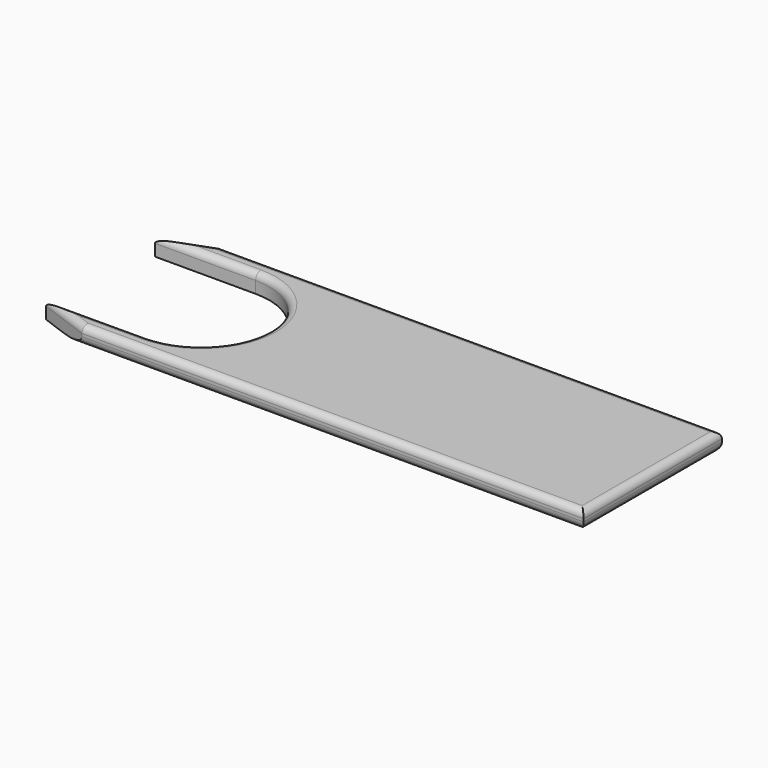
from build123d import *

# Parameters (mm, degrees)
F0_W         = 60
F0_H         = 18.8
F2_DEPTH     = 2
F3_DEPTH     = 3
F5_T1_DEPTH  = 30.5361420581
F6_SIZE2     = 5.494945
F6_SIZE      = 1.99999
F7_T1_DEPTH  = 59.3887824638
F7_T3_DEPTH  = 59.3938374638
F7_T5_DEPTH  = 22.4213203436
F7_T7_DEPTH  = 10.7363912706
F7_T9_DEPTH  = 3.6213303413
F7_T11_DEPTH = 12.745712209
F7_T13_DEPTH = 10.7363785984
F7_T15_DEPTH = 12.740667054
F7_T18_ANGLE = 180
F8_R         = 0.9656854249


# Not quite as in the source:
# - a fillet or chamfer that OpenCascade refuses, or shapes differently, is made with other operations: its cross-section is extruded or revolved along the edge and cut away or added
# - a fillet or chamfer is up to 0.001 mm smaller than in the source, because OpenCascade refuses the exact size


with BuildPart() as f2:
    # F0 (on Top) → F2 (new body)
    with BuildSketch(Plane.XY):
        Rectangle(F0_W, F0_H)
    extrude(amount=F2_DEPTH)


with BuildPart() as f3:
    # F1 (on Top) → F3 (new body)
    with BuildSketch(Plane.XY):
        with BuildLine():
            ThreePointArc((-19.0649479628, -7.3999999978), (-13.832357782, -5.2325901785), (-11.6649479628, 2.2e-09))
            ThreePointArc((-11.6649479628, 2.2e-09), (-13.832357782, 5.232590183), (-19.0649479628, 7.4000000022))
            Line((-19.0649479628, 7.4000000022), (-19.0649479628, -7.3999999978))
        make_face()
        with BuildLine():
            Line((-19.0649479628, -7.3999999978), (-19.0649479628, 7.4000000022))
            ThreePointArc((-19.0649479628, 7.4000000022), (-26.4649479628, 2.2e-09), (-19.0649479628, -7.3999999978))
        make_face()
        with BuildLine():
            ThreePointArc((-19.0649479628, -7.3999999978), (-26.4649479628, 2.2e-09), (-19.0649479628, 7.4000000022))
            Line((-19.0649479628, 7.4000000022), (-58.9926913381, 7.4000000022))
            Line((-58.9926913381, 7.4000000022), (-58.9926913381, -7.3999999978))
            Line((-58.9926913381, -7.3999999978), (-19.0649479628, -7.3999999978))
        make_face()
    extrude(amount=F3_DEPTH)


with BuildPart() as f2_1:
    add(f2.part)

    # F4: cut F3
    add(f3.part, mode=Mode.SUBTRACT)

    # F5: chamfer of 5.5 x 2.0018362885 on 1 edges, made by hand

    # F5_s2 → F5_t1 (cut)
    with BuildSketch(Plane.XY.offset(-14.268071029)):
        Polygon((-24.5, -9.4), (-30, -7.3981637115), (-30, -9.4), align=None)
    extrude(amount=F5_T1_DEPTH, mode=Mode.SUBTRACT)

    # F6 (size 2 and 5.4949548389 in the source; OpenCascade refuses exactly that, so slightly less here)
    f6_edges = [f2_1.edges().sort_by_distance(p)[0] for p in [
        (-30, 9.4, 1),
    ]]
    f6_side = f2_1.faces().sort_by_distance((-30, 8.4, 1))[0]
    chamfer(f6_edges, length=F6_SIZE, length2=F6_SIZE2, reference=f6_side)

    # F7: fillet of radius 0.7242640687 on 9 edges, made by hand

    # F7_s2 → F7_t1 (cut)
    with BuildSketch(Plane.YZ.offset(-27.578122292)):
        with BuildLine():
            ThreePointArc((-8.6757359313, 2), (-9.1878679656, 1.7878679656), (-9.4, 1.2757359313))
            Line((-9.4, 1.2757359313), (-9.4, 2))
            Line((-9.4, 2), (-8.6757359313, 2))
        make_face()
    extrude(amount=F7_T1_DEPTH, mode=Mode.SUBTRACT)

    # F7_s4 → F7_t3 (cut)
    with BuildSketch(Plane.YZ.offset(-27.583177292)):
        with BuildLine():
            ThreePointArc((9.4, 1.2757359313), (9.1878679656, 1.7878679656), (8.6757359313, 2))
            Line((8.6757359313, 2), (9.4, 2))
            Line((9.4, 2), (9.4, 1.2757359313))
        make_face()
    extrude(amount=F7_T3_DEPTH, mode=Mode.SUBTRACT)

    # F7_s6 → F7_t5 (cut)
    with BuildSketch(Plane.XZ.offset(-11.2106601718)):
        with BuildLine():
            ThreePointArc((30, 1.2757359313), (29.7878679656, 1.7878679656), (29.2757359313, 2))
            Line((29.2757359313, 2), (30, 2))
            Line((30, 2), (30, 1.2757359313))
        make_face()
    extrude(amount=F7_T5_DEPTH, mode=Mode.SUBTRACT)

    # F7_s8 → F7_t7 (cut)
    with BuildSketch(Plane(origin=(-25.8093615097, 9.3938393551, 0), x_dir=(0, 0, 1), z_dir=(0.9396926208, -0.3420201433, 0))):
        with BuildLine():
            ThreePointArc((2, 16.4883400783), (1.7878679656, 17.0004721126), (1.2757359313, 17.212604147))
            Line((1.2757359313, 17.212604147), (2, 17.212604147))
            Line((2, 17.212604147), (2, 16.4883400783))
        make_face()
    extrude(amount=F7_T7_DEPTH, mode=Mode.SUBTRACT)

    # F7_s10 → F7_t9 (cut)
    with BuildSketch(Plane.XZ.offset(-9.2106701718)):
        with BuildLine():
            ThreePointArc((-29.2757359313, 2), (-29.7878679656, 1.7878679656), (-30, 1.2757359313))
            Line((-30, 1.2757359313), (-30, 2))
            Line((-30, 2), (-29.2757359313, 2))
        make_face()
    extrude(amount=F7_T9_DEPTH, mode=Mode.SUBTRACT)

    # F7_s12 → F7_t11 (cut)
    with BuildSketch(Plane.YZ.offset(-31.8106601718)):
        with BuildLine():
            ThreePointArc((8.1242640709, 2), (7.6121320366, 1.7878679656), (7.4000000022, 1.2757359313))
            Line((7.4000000022, 1.2757359313), (7.4000000022, 2))
            Line((7.4000000022, 2), (8.1242640709, 2))
        make_face()
    extrude(amount=F7_T11_DEPTH, mode=Mode.SUBTRACT)

    # F7_s14 → F7_t13 (cut)
    with BuildSketch(Plane(origin=(-25.8138396564, -9.3954391126, 0), x_dir=(0, 0, 1), z_dir=(0.9396929736, 0.342019174, 0))):
        with BuildLine():
            ThreePointArc((1.2757359313, -17.2143126223), (1.7878679656, -17.0021805879), (2, -16.4900485536))
            Line((2, -16.4900485536), (2, -17.2143126223))
            Line((2, -17.2143126223), (1.2757359313, -17.2143126223))
        make_face()
    extrude(amount=F7_T13_DEPTH, mode=Mode.SUBTRACT)

    # F7_s16 → F7_t15 (cut)
    with BuildSketch(Plane.YZ.offset(-31.8056150167)):
        with BuildLine():
            ThreePointArc((-8.1242640665, 2), (-7.6121320321, 1.7878679656), (-7.3999999978, 1.2757359313))
            Line((-7.3999999978, 1.2757359313), (-7.3999999978, 2))
            Line((-7.3999999978, 2), (-8.1242640665, 2))
        make_face()
    extrude(amount=F7_T15_DEPTH, mode=Mode.SUBTRACT)

    # F7_s17 → F7_t18 (revolve, cut)
    with BuildSketch(Plane.YZ.offset(-19.0649479628)):
        with BuildLine():
            ThreePointArc((8.1242640709, 2), (7.6121320366, 1.7878679656), (7.4000000022, 1.2757359313))
            Line((7.4000000022, 1.2757359313), (7.4000000022, 2))
            Line((7.4000000022, 2), (8.1242640709, 2))
        make_face()
    revolve(axis=Axis((-19.0649479628, 2.2e-09, 2), (0, 0, -1)), revolution_arc=F7_T18_ANGLE, mode=Mode.SUBTRACT)

    # F8
    f8_edges = [f2_1.edges().sort_by_distance(p)[0] for p in [
        (2.75, -9.4, 0),
        (30, 0, 0),
        (2.747473, 9.4, 0),
    ]]
    fillet(f8_edges, radius=F8_R)


solid = f2_1.part
